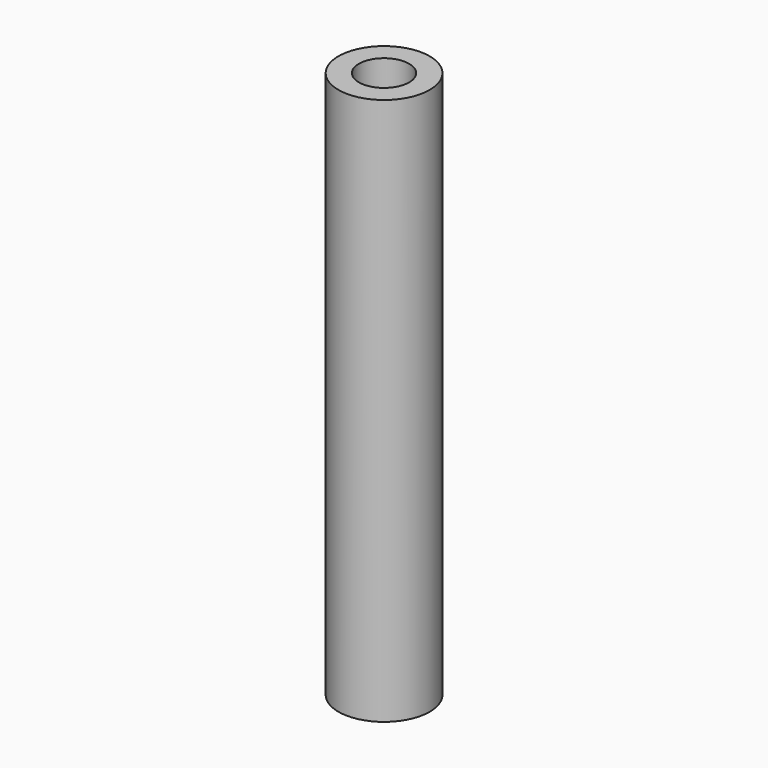
from build123d import *

# Parameters (mm, degrees)
F0_R     = 12.7
F1_DEPTH = 152.4
F3_D     = 14
F3_DEPTH = 50.8
F3_TIP   = 4.2060243332


# Not quite as in the source:
# - a feature of the source that left no trace in its solid (it failed there, or was rolled back) is left out


with BuildPart() as f1:
    # F0 (on Top) → F1 (new body)
    with BuildSketch(Plane.XY):
        Circle(F0_R)
    extrude(amount=F1_DEPTH)

    # F3
    with Locations(Plane.XY.offset(152.4)):
        with Locations((0, 0)):
            Hole(F3_D / 2, depth=F3_DEPTH)
            with Locations((0, 0, -(F3_DEPTH + F3_TIP / 2))):  # 118° drill point
                Cone(0, F3_D / 2, F3_TIP, mode=Mode.SUBTRACT)


solid = f1.part
